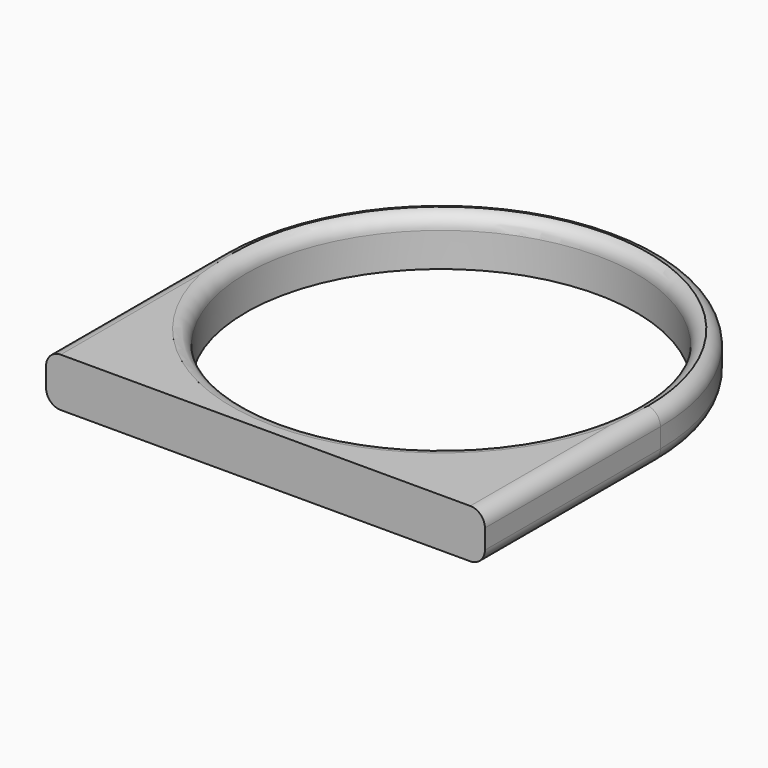
from build123d import *

# Parameters (mm, degrees)
F1_DEPTH    = 10
F2_T1_DEPTH = 52.5
F2_T6_ANGLE = 180
F2_T8_ANGLE = 180


# Not quite as in the source:
# - a fillet or chamfer that OpenCascade refuses, or shapes differently, is made with other operations: its cross-section is extruded or revolved along the edge and cut away or added


with BuildPart() as f1:
    # F0 (on Top) → F1 (new body)
    with BuildSketch(Plane.XY):
        with BuildLine():
            Line((45, -45), (45, 0))
            ThreePointArc((45, 0), (0, 45), (-45, 0))
            Line((-45, 0), (-45, -45))
            Line((-45, -45), (0, -45))
            Line((0, -45), (45, -45))
        make_face()
        with BuildLine():
            ThreePointArc((0, 40), (40, 0), (0, -40))
            ThreePointArc((0, -40), (-40, 0), (0, 40))
        make_face(mode=Mode.SUBTRACT)
    extrude(amount=F1_DEPTH)

    # F2: fillet of radius 3 on 6 edges, made by hand

    # F2_s2 → F2_t1 (cut)
    with BuildSketch(Plane.XZ):
        with BuildLine():
            ThreePointArc((-42, 10), (-44.1213203436, 9.1213203436), (-45, 7))
            Line((-45, 7), (-45, 10))
            Line((-45, 10), (-42, 10))
        make_face()
        with BuildLine():
            ThreePointArc((-45, 3), (-44.1213203436, 0.8786796564), (-42, 0))
            Line((-42, 0), (-45, 0))
            Line((-45, 0), (-45, 3))
        make_face()
        with BuildLine():
            ThreePointArc((45, 3), (44.1213203436, 0.8786796564), (42, 0))
            Line((42, 0), (45, 0))
            Line((45, 0), (45, 3))
        make_face()
        with BuildLine():
            ThreePointArc((45, 7), (44.1213203436, 9.1213203436), (42, 10))
            Line((42, 10), (45, 10))
            Line((45, 10), (45, 7))
        make_face()
    extrude(amount=F2_T1_DEPTH, mode=Mode.SUBTRACT)

    # F2_s3 → F2_t4 (revolve, cut)
    with BuildSketch(Plane.YZ):
        with BuildLine():
            ThreePointArc((43, 10), (40.8786796564, 9.1213203436), (40, 7))
            Line((40, 7), (40, 10))
            Line((40, 10), (43, 10))
        make_face()
    revolve(axis=Axis((0, 0, 10), (0, 0, 1)), mode=Mode.SUBTRACT)

    # F2_s5 → F2_t6 (revolve, cut)
    with BuildSketch(Plane.XZ):
        with BuildLine():
            ThreePointArc((42, 10), (44.1213203436, 9.1213203436), (45, 7))
            Line((45, 7), (45, 10))
            Line((45, 10), (42, 10))
        make_face()
    revolve(axis=Axis((0, 0, 10), (0, 0, 1)), revolution_arc=F2_T6_ANGLE, mode=Mode.SUBTRACT)

    # F2_s7 → F2_t8 (revolve, cut)
    with BuildSketch(Plane.XZ):
        with BuildLine():
            ThreePointArc((42, 0), (44.1213203436, 0.8786796564), (45, 3))
            Line((45, 3), (45, 0))
            Line((45, 0), (42, 0))
        make_face()
    revolve(axis=Axis((0, 0, 0), (0, 0, 1)), revolution_arc=F2_T8_ANGLE, mode=Mode.SUBTRACT)


solid = f1.part
